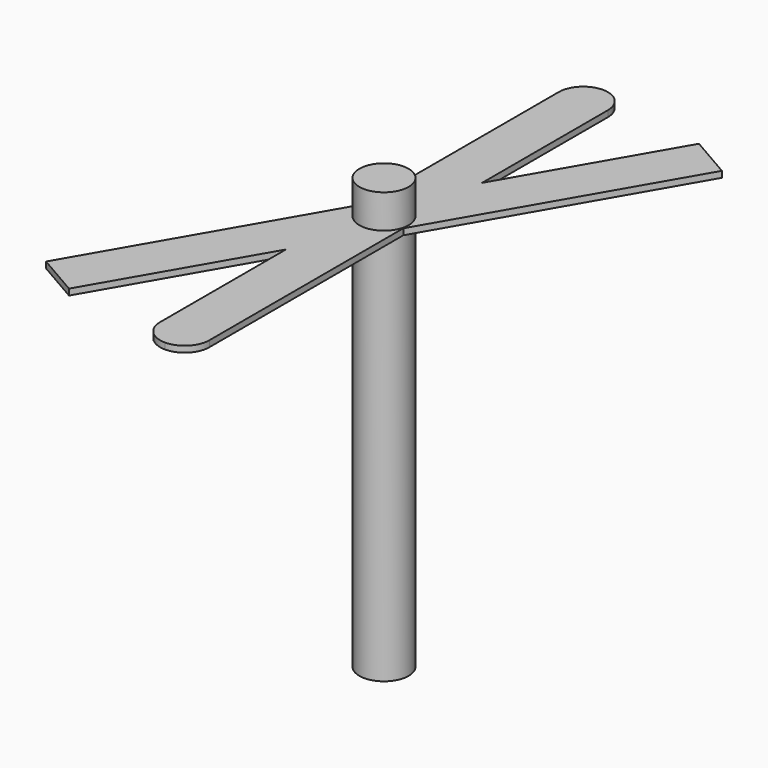
from build123d import *

# Parameters (mm, degrees)
F0_W     = 12.7
F0_H     = 222.25
F3_W     = 25.4
F3_H     = 3.175
F4_DEPTH = 141.2875
F6_R     = 12.69999
F8_W     = 25.4
F8_H     = 3.175
F9_DEPTH = 141.2875


# Not quite as in the source:
# - a fillet or chamfer is up to 0.001 mm smaller than in the source, because OpenCascade refuses the exact size


with BuildPart() as f1:
    # F0 (on Front) → F1 (revolve)
    with BuildSketch(Plane.XZ):
        with Locations((-6.35, -16.2413566351)):
            Rectangle(F0_W, F0_H)
    revolve(axis=Axis((0, 0, -16.2413566351), (0, 0, -1)))

    # F3 (on Front) → F4 (join, symmetric)
    with BuildSketch(Plane.XZ):
        with Locations((0, 75.8653144777)):
            Rectangle(F3_W, F3_H)
    extrude(amount=F4_DEPTH, both=True)

    # F6 (radius 12.7 in the source; OpenCascade refuses exactly that, so slightly less here)
    f6_edges = [f1.edges().sort_by_distance(p)[0] for p in [
        (12.7, 141.2875, 75.865314),
        (-12.7, 141.2875, 75.865314),
        (-12.7, -141.2875, 75.865314),
        (12.7, -141.2875, 75.865314),
    ]]
    fillet(f6_edges, radius=F6_R)

    # F8 (on line) → F9 (join, symmetric)
    with BuildSketch(Plane(origin=(0, 0, 0), x_dir=(-0.8660254038, 0.5, 0), z_dir=(0.5, 0.8660254038, 0))):
        with Locations((0, 75.8653144777)):
            Rectangle(F8_W, F8_H)
    extrude(amount=F9_DEPTH, both=True)


solid = f1.part
